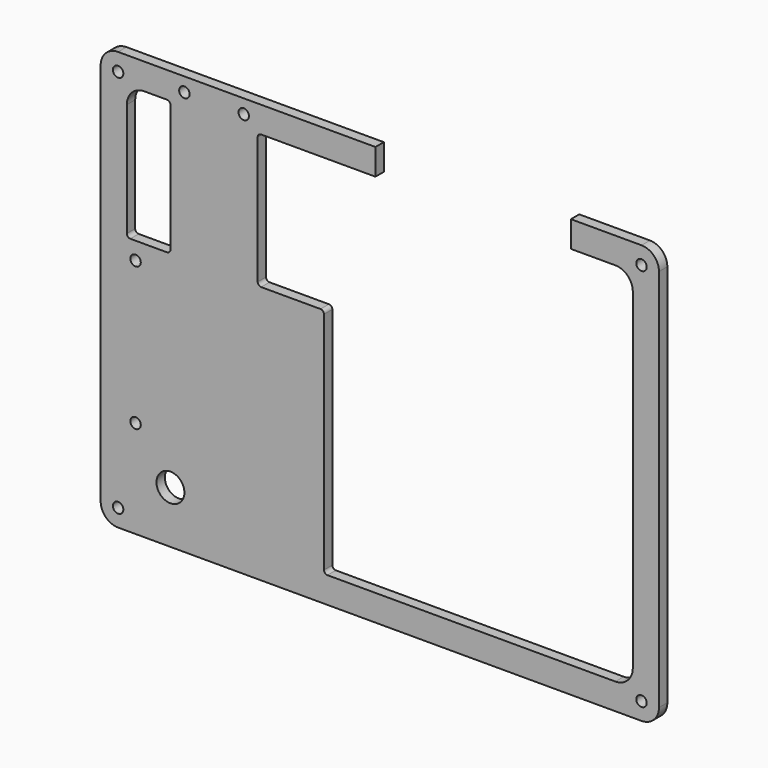
from build123d import *

# Parameters (mm, degrees)
F1_DEPTH  = 3
F2_R      = 1.5
F3_DEPTH  = 25
F5_DEPTH  = 3
F7_D      = 3
F7_DEPTH  = 3
F7_TIP    = 0.9012909285
F8_DEPTH  = 3
F9_R      = 1.5
F9_R_2    = 4
F10_DEPTH = 25


# Not quite as in the source:
# - a feature names something its author has since deleted; it is built from what else it names


with BuildPart() as f1:
    # F0 (on Front) → F1 (new body)
    with BuildSketch(Plane.XZ):
        with BuildLine():
            Line((-75, -60), (75, -60))
            ThreePointArc((75, -60), (78.5355339059, -58.5355339059), (80, -55))
            Line((80, -55), (80, 55))
            ThreePointArc((80, 55), (78.5355339059, 58.5355339059), (75, 60))
            Line((75, 60), (-75, 60))
            ThreePointArc((-75, 60), (-78.5355339059, 58.5355339059), (-80, 55))
            Line((-80, 55), (-80, -55))
            ThreePointArc((-80, -55), (-78.5355339059, -58.5355339059), (-75, -60))
        make_face()
    extrude(amount=F1_DEPTH)

    # F2 (on Front) → F3 (cut)
    with BuildSketch(Plane.XZ):
        with Locations((-75, 55)):
            Circle(F2_R)
        with Locations((75, 55)):
            Circle(F2_R)
        with Locations((75, -55)):
            Circle(F2_R)
        with Locations((-75, -55)):
            Circle(F2_R)
    extrude(amount=F3_DEPTH, mode=Mode.SUBTRACT)

    # F4 (on face) → F5 (cut)
    with BuildSketch(Plane.XZ.offset(3)):
        with BuildLine():
            ThreePointArc((72.5, 47.5), (71.0355339059, 51.0355339059), (67.5, 52.5))
            Line((67.5, 52.5), (54.75, 52.5))
            Line((54.75, 52.5), (54.75, 60))
            Line((54.75, 60), (-1.25, 60))
            Line((-1.25, 60), (-1.25, 52.5))
            Line((-1.25, 52.5), (-34, 52.5))
            ThreePointArc((-34, 52.5), (-34.7071067812, 52.2071067812), (-35, 51.5))
            Line((-35, 51.5), (-35, 15))
            ThreePointArc((-35, 15), (-34.7071067812, 14.2928932188), (-34, 14))
            Line((-34, 14), (-17, 14))
            ThreePointArc((-17, 14), (-16.2928932188, 13.7071067812), (-16, 13))
            Line((-16, 13), (-16, -51.5))
            ThreePointArc((-16, -51.5), (-15.7071067812, -52.2071067812), (-15, -52.5))
            Line((-15, -52.5), (67.5, -52.5))
            ThreePointArc((67.5, -52.5), (71.0355339059, -51.0355339059), (72.5, -47.5))
            Line((72.5, -47.5), (72.5, 47.5))
        make_face()
    extrude(amount=-F5_DEPTH, mode=Mode.SUBTRACT)

    # F7
    with Locations(Plane.XZ.offset(3)):
        with Locations((-56, 56), (-39, 56)):
            Hole(F7_D / 2, depth=F7_DEPTH)
            with Locations((0, 0, -(F7_DEPTH + F7_TIP / 2))):  # 118° drill point
                Cone(0, F7_D / 2, F7_TIP, mode=Mode.SUBTRACT)

    # F4 (on face) → F8 (cut)
    with BuildSketch(Plane.XZ.offset(3)):
        with BuildLine():
            ThreePointArc((72.5, 47.5), (71.0355339059, 51.0355339059), (67.5, 52.5))
            Line((67.5, 52.5), (54.75, 52.5))
            Line((54.75, 52.5), (54.75, 60))
            Line((54.75, 60), (-1.25, 60))
            Line((-1.25, 60), (-1.25, 52.5))
            Line((-1.25, 52.5), (-34, 52.5))
            ThreePointArc((-34, 52.5), (-34.7071067812, 52.2071067812), (-35, 51.5))
            Line((-35, 51.5), (-35, 15))
            ThreePointArc((-35, 15), (-34.7071067812, 14.2928932188), (-34, 14))
            Line((-34, 14), (-17, 14))
            ThreePointArc((-17, 14), (-16.2928932188, 13.7071067812), (-16, 13))
            Line((-16, 13), (-16, -51.5))
            ThreePointArc((-16, -51.5), (-15.7071067812, -52.2071067812), (-15, -52.5))
            Line((-15, -52.5), (67.5, -52.5))
            ThreePointArc((67.5, -52.5), (71.0355339059, -51.0355339059), (72.5, -47.5))
            Line((72.5, -47.5), (72.5, 47.5))
        make_face()
        with BuildLine():
            ThreePointArc((-67.5, 52.5), (-71.0355339059, 51.0355339059), (-72.5, 47.5))
            Line((-72.5, 47.5), (-72.5, 15))
            ThreePointArc((-72.5, 15), (-72.2071067812, 14.2928932188), (-71.5, 14))
            Line((-71.5, 14), (-61, 14))
            ThreePointArc((-61, 14), (-60.2928932188, 14.2928932188), (-60, 15))
            Line((-60, 15), (-60, 51.5))
            ThreePointArc((-60, 51.5), (-60.2928932188, 52.2071067812), (-61, 52.5))
            Line((-61, 52.5), (-67.5, 52.5))
        make_face()
    extrude(amount=-F8_DEPTH, mode=Mode.SUBTRACT)

    # F9 (on face) → F10 (cut)
    with BuildSketch(Plane.XZ.offset(3)):
        with Locations((-70, 9)):
            Circle(F9_R)
        with Locations((-60, -45)):
            Circle(F9_R_2)
        with Locations((-70, -32)):
            Circle(F9_R)
    extrude(amount=-F10_DEPTH, mode=Mode.SUBTRACT)


solid = f1.part
